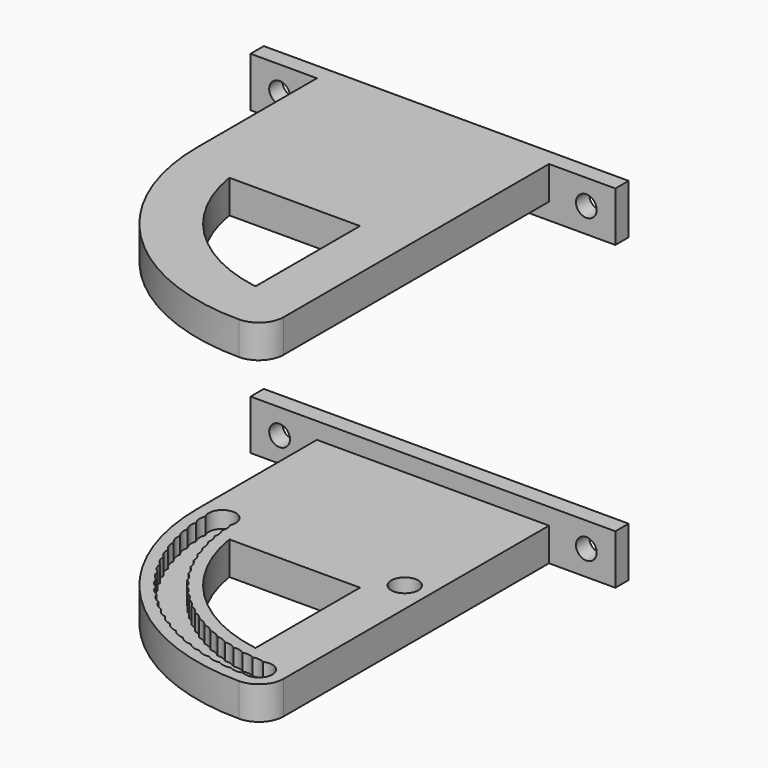
from build123d import *

# Parameters (mm, degrees)
F0_R          = 1.625
F1_DEPTH      = 2
F2_R          = 1.625
F3_DEPTH      = 2
F4_W          = 8
F4_H          = 2
F4_W_2        = 28
F5_DEPTH      = 2
F5_DEPTH_BACK = 4
F6_R          = 1.25
F7_DEPTH      = 25


with BuildPart() as f1:
    # F0 (on Top) → F1 (new body)
    with BuildSketch(Plane.XY):
        with BuildLine():
            Line((-25, 20), (-25, 0))
            ThreePointArc((-25, 0), (-17.6776695297, -17.6776695297), (0, -25))
            ThreePointArc((0, -25), (2.1213203436, -24.1213203436), (3, -22))
            Line((3, -22), (3, 20))
            Line((3, 20), (-25, 20))
        make_face()
        with BuildLine():
            ThreePointArc((-0.6717668116, -20.520353302), (1.6241299546, -22.0531685096), (-0.7671020315, -23.4325430092))
            ThreePointArc((-0.7671020315, -23.4325430092), (-1.5451489281, -23.5744170615), (-2.2980212458, -23.3322012626))
            ThreePointArc((-2.2980212458, -23.3322012626), (-3.0836812912, -23.42288485), (-3.8190999803, -23.1319474482))
            ThreePointArc((-3.8190999803, -23.1319474482), (-4.6090088576, -23.1710522495), (-5.3238247424, -22.8326390835))
            ThreePointArc((-5.3238247424, -22.8326390835), (-6.1145999405, -22.8199976461), (-6.8057520696, -22.435557853))
            ThreePointArc((-6.8057520696, -22.435557853), (-7.5940073678, -22.3712243093), (-8.2585361216, -21.9424041193))
            ThreePointArc((-8.2585361216, -21.9424041193), (-9.0408960896, -21.8266539556), (-9.675955854, -21.3552896425))
            ThreePointArc((-9.675955854, -21.3552896425), (-10.4490703064, -21.1886185187), (-11.0519416581, -20.676728537))
            ThreePointArc((-11.0519416581, -20.676728537), (-11.8125, -20.4598501644), (-12.3806013512, -19.9096265055))
            ThreePointArc((-12.3806013512, -19.9096265055), (-13.1253467551, -19.6434695906), (-13.6562454086, -19.0572683968))
            ThreePointArc((-13.6562454086, -19.0572683968), (-14.3819887603, -18.7429726644), (-14.8734113266, -18.123304139))
            ThreePointArc((-14.8734113266, -18.123304139), (-15.5770448817, -17.7622154517), (-16.026887014, -17.1117331106))
            ThreePointArc((-16.026887014, -17.1117331106), (-16.7053977055, -16.7053977055), (-17.1117331106, -16.026887014))
            ThreePointArc((-17.1117331106, -16.026887014), (-17.7622154517, -15.5770448817), (-18.123304139, -14.8734113266))
            ThreePointArc((-18.123304139, -14.8734113266), (-18.7429726644, -14.3819887603), (-19.0572683968, -13.6562454086))
            ThreePointArc((-19.0572683968, -13.6562454086), (-19.6434695906, -13.1253467551), (-19.9096265055, -12.3806013512))
            ThreePointArc((-19.9096265055, -12.3806013512), (-20.4598501644, -11.8125), (-20.676728537, -11.0519416581))
            ThreePointArc((-20.676728537, -11.0519416581), (-21.1886185187, -10.4490703064), (-21.3552896425, -9.675955854))
            ThreePointArc((-21.3552896425, -9.675955854), (-21.8266539556, -9.0408960896), (-21.9424041193, -8.2585361216))
            ThreePointArc((-21.9424041193, -8.2585361216), (-22.3712243093, -7.5940073678), (-22.435557853, -6.8057520696))
            ThreePointArc((-22.435557853, -6.8057520696), (-22.8199976461, -6.1145999405), (-22.8326390835, -5.3238247424))
            ThreePointArc((-22.8326390835, -5.3238247424), (-23.1710522495, -4.6090088576), (-23.1319474482, -3.8190999803))
            ThreePointArc((-23.1319474482, -3.8190999803), (-23.42288485, -3.0836812912), (-23.3322012626, -2.2980212458))
            ThreePointArc((-23.3322012626, -2.2980212458), (-23.5744170615, -1.5451489281), (-23.4325430092, -0.7671020315))
            ThreePointArc((-23.4325430092, -0.7671020315), (-22.0531685096, 1.6241299546), (-20.520353302, -0.6717668116))
            ThreePointArc((-20.520353302, -0.6717668116), (-20.331375561, -1.3325887581), (-20.4324819988, -2.0124238261))
            ThreePointArc((-20.4324819988, -2.0124238261), (-20.2006890505, -2.6594711665), (-20.2571156709, -3.3444633329))
            ThreePointArc((-20.2571156709, -3.3444633329), (-19.9835000882, -3.9749653111), (-19.9950052637, -4.6621813342))
            ThreePointArc((-19.9950052637, -4.6621813342), (-19.6807387106, -5.273438044), (-19.6472731743, -5.9599351593))
            ThreePointArc((-19.6472731743, -5.9599351593), (-19.2937013885, -6.5493291056), (-19.2154084448, -7.2321676271))
            ThreePointArc((-19.2154084448, -7.2321676271), (-18.8240454749, -7.7971749344), (-18.7012603864, -8.4734308428))
            ThreePointArc((-18.7012603864, -8.4734308428), (-18.2737821087, -9.0116320632), (-18.10703066, -9.6784095268))
            ThreePointArc((-18.10703066, -9.6784095268), (-17.6452676021, -10.1875), (-17.4352638484, -10.8419437753))
            ThreePointArc((-17.4352638484, -10.8419437753), (-16.9411933507, -11.3197434978), (-16.6888365603, -11.959051156))
            ThreePointArc((-16.6888365603, -11.959051156), (-16.1645743084, -12.4035141161), (-15.8709451119, -13.0249480438))
            ThreePointArc((-15.8709451119, -13.0249480438), (-15.3187360774, -13.4341709827), (-14.98509184, -14.0350701044))
            ThreePointArc((-14.98509184, -14.0350701044), (-14.4073006667, -14.4073006667), (-14.0350701044, -14.98509184))
            ThreePointArc((-14.0350701044, -14.98509184), (-13.4341709827, -15.3187360774), (-13.0249480438, -15.8709451119))
            ThreePointArc((-13.0249480438, -15.8709451119), (-12.4035141161, -16.1645743084), (-11.959051156, -16.6888365603))
            ThreePointArc((-11.959051156, -16.6888365603), (-11.3197434978, -16.9411933507), (-10.8419437753, -17.4352638484))
            ThreePointArc((-10.8419437753, -17.4352638484), (-10.1875, -17.6452676021), (-9.6784095268, -18.10703066))
            ThreePointArc((-9.6784095268, -18.10703066), (-9.0116320632, -18.2737821087), (-8.4734308428, -18.7012603864))
            ThreePointArc((-8.4734308428, -18.7012603864), (-7.7971749344, -18.8240454749), (-7.2321676271, -19.2154084448))
            ThreePointArc((-7.2321676271, -19.2154084448), (-6.5493291056, -19.2937013885), (-5.9599351593, -19.6472731743))
            ThreePointArc((-5.9599351593, -19.6472731743), (-5.273438044, -19.6807387106), (-4.6621813342, -19.9950052637))
            ThreePointArc((-4.6621813342, -19.9950052637), (-3.9749653111, -19.9835000882), (-3.3444633329, -20.2571156709))
            ThreePointArc((-3.3444633329, -20.2571156709), (-2.6594711665, -20.2006890505), (-2.0124238261, -20.4324819988))
            ThreePointArc((-2.0124238261, -20.4324819988), (-1.3325887581, -20.331375561), (-0.6717668116, -20.520353302))
        make_face(mode=Mode.SUBTRACT)
        with BuildLine():
            ThreePointArc((-3, -18.7616630393), (-13.4350288425, -13.4350288425), (-18.7616630393, -3))
            Line((-18.7616630393, -3), (-3, -3))
            Line((-3, -3), (-3, -18.7616630393))
        make_face(mode=Mode.SUBTRACT)
        Circle(F0_R, mode=Mode.SUBTRACT)
    extrude(amount=F1_DEPTH)

    # F2 (on face) → F3 (join)
    with BuildSketch(Plane(origin=(0, 0, 0), x_dir=(1, 0, 0), z_dir=(0, 0, -1))):
        with BuildLine():
            ThreePointArc((0, 25), (-17.6776695297, 17.6776695297), (-25, 0))
            Line((-25, 0), (-25, -20))
            Line((-25, -20), (3, -20))
            Line((3, -20), (3, 22))
            ThreePointArc((3, 22), (2.1213203436, 24.1213203436), (0, 25))
        make_face()
        Circle(F2_R, mode=Mode.SUBTRACT)
        with BuildLine():
            Line((-3, 18.7616630393), (-3, 3))
            Line((-3, 3), (-18.7616630393, 3))
            ThreePointArc((-18.7616630393, 3), (-13.4350288425, 13.4350288425), (-3, 18.7616630393))
        make_face(mode=Mode.SUBTRACT)
        with BuildLine():
            ThreePointArc((-2.2980212458, 23.3322012626), (-1.5451489281, 23.5744170615), (-0.7671020315, 23.4325430092))
            ThreePointArc((-0.7671020315, 23.4325430092), (1.6241299546, 22.0531685096), (-0.6717668116, 20.520353302))
            ThreePointArc((-0.6717668116, 20.520353302), (-1.3325887581, 20.331375561), (-2.0124238261, 20.4324819988))
            ThreePointArc((-2.0124238261, 20.4324819988), (-2.6594711665, 20.2006890505), (-3.3444633329, 20.2571156709))
            ThreePointArc((-3.3444633329, 20.2571156709), (-3.9749653111, 19.9835000882), (-4.6621813342, 19.9950052637))
            ThreePointArc((-4.6621813342, 19.9950052637), (-5.273438044, 19.6807387106), (-5.9599351593, 19.6472731743))
            ThreePointArc((-5.9599351593, 19.6472731743), (-6.5493291056, 19.2937013885), (-7.2321676271, 19.2154084448))
            ThreePointArc((-7.2321676271, 19.2154084448), (-7.7971749344, 18.8240454749), (-8.4734308428, 18.7012603864))
            ThreePointArc((-8.4734308428, 18.7012603864), (-9.0116320632, 18.2737821087), (-9.6784095268, 18.10703066))
            ThreePointArc((-9.6784095268, 18.10703066), (-10.1875, 17.6452676021), (-10.8419437753, 17.4352638484))
            ThreePointArc((-10.8419437753, 17.4352638484), (-11.3197434978, 16.9411933507), (-11.959051156, 16.6888365603))
            ThreePointArc((-11.959051156, 16.6888365603), (-12.4035141161, 16.1645743084), (-13.0249480438, 15.8709451119))
            ThreePointArc((-13.0249480438, 15.8709451119), (-13.4341709827, 15.3187360774), (-14.0350701044, 14.98509184))
            ThreePointArc((-14.0350701044, 14.98509184), (-14.4073006667, 14.4073006667), (-14.98509184, 14.0350701044))
            ThreePointArc((-14.98509184, 14.0350701044), (-15.3187360774, 13.4341709827), (-15.8709451119, 13.0249480438))
            ThreePointArc((-15.8709451119, 13.0249480438), (-16.1645743084, 12.4035141161), (-16.6888365603, 11.959051156))
            ThreePointArc((-16.6888365603, 11.959051156), (-16.9411933507, 11.3197434978), (-17.4352638484, 10.8419437753))
            ThreePointArc((-17.4352638484, 10.8419437753), (-17.6452676021, 10.1875), (-18.10703066, 9.6784095268))
            ThreePointArc((-18.10703066, 9.6784095268), (-18.2737821087, 9.0116320632), (-18.7012603864, 8.4734308428))
            ThreePointArc((-18.7012603864, 8.4734308428), (-18.8240454749, 7.7971749344), (-19.2154084448, 7.2321676271))
            ThreePointArc((-19.2154084448, 7.2321676271), (-19.2937013885, 6.5493291056), (-19.6472731743, 5.9599351593))
            ThreePointArc((-19.6472731743, 5.9599351593), (-19.6807387106, 5.273438044), (-19.9950052637, 4.6621813342))
            ThreePointArc((-19.9950052637, 4.6621813342), (-19.9835000882, 3.9749653111), (-20.2571156709, 3.3444633329))
            ThreePointArc((-20.2571156709, 3.3444633329), (-20.2006890505, 2.6594711665), (-20.4324819988, 2.0124238261))
            ThreePointArc((-20.4324819988, 2.0124238261), (-20.331375561, 1.3325887581), (-20.520353302, 0.6717668116))
            ThreePointArc((-20.520353302, 0.6717668116), (-22.0531685096, -1.6241299546), (-23.4325430092, 0.7671020315))
            ThreePointArc((-23.4325430092, 0.7671020315), (-23.5744170615, 1.5451489281), (-23.3322012626, 2.2980212458))
            ThreePointArc((-23.3322012626, 2.2980212458), (-23.42288485, 3.0836812912), (-23.1319474482, 3.8190999803))
            ThreePointArc((-23.1319474482, 3.8190999803), (-23.1710522495, 4.6090088576), (-22.8326390835, 5.3238247424))
            ThreePointArc((-22.8326390835, 5.3238247424), (-22.8199976461, 6.1145999405), (-22.435557853, 6.8057520696))
            ThreePointArc((-22.435557853, 6.8057520696), (-22.3712243093, 7.5940073678), (-21.9424041193, 8.2585361216))
            ThreePointArc((-21.9424041193, 8.2585361216), (-21.8266539556, 9.0408960896), (-21.3552896425, 9.675955854))
            ThreePointArc((-21.3552896425, 9.675955854), (-21.1886185187, 10.4490703064), (-20.676728537, 11.0519416581))
            ThreePointArc((-20.676728537, 11.0519416581), (-20.4598501644, 11.8125), (-19.9096265055, 12.3806013512))
            ThreePointArc((-19.9096265055, 12.3806013512), (-19.6434695906, 13.1253467551), (-19.0572683968, 13.6562454086))
            ThreePointArc((-19.0572683968, 13.6562454086), (-18.7429726644, 14.3819887603), (-18.123304139, 14.8734113266))
            ThreePointArc((-18.123304139, 14.8734113266), (-17.7622154517, 15.5770448817), (-17.1117331106, 16.026887014))
            ThreePointArc((-17.1117331106, 16.026887014), (-16.7053977055, 16.7053977055), (-16.026887014, 17.1117331106))
            ThreePointArc((-16.026887014, 17.1117331106), (-15.5770448817, 17.7622154517), (-14.8734113266, 18.123304139))
            ThreePointArc((-14.8734113266, 18.123304139), (-14.3819887603, 18.7429726644), (-13.6562454086, 19.0572683968))
            ThreePointArc((-13.6562454086, 19.0572683968), (-13.1253467551, 19.6434695906), (-12.3806013512, 19.9096265055))
            ThreePointArc((-12.3806013512, 19.9096265055), (-11.8125, 20.4598501644), (-11.0519416581, 20.676728537))
            ThreePointArc((-11.0519416581, 20.676728537), (-10.4490703064, 21.1886185187), (-9.675955854, 21.3552896425))
            ThreePointArc((-9.675955854, 21.3552896425), (-9.0408960896, 21.8266539556), (-8.2585361216, 21.9424041193))
            ThreePointArc((-8.2585361216, 21.9424041193), (-7.5940073678, 22.3712243093), (-6.8057520696, 22.435557853))
            ThreePointArc((-6.8057520696, 22.435557853), (-6.1145999405, 22.8199976461), (-5.3238247424, 22.8326390835))
            ThreePointArc((-5.3238247424, 22.8326390835), (-4.6090088576, 23.1710522495), (-3.8190999803, 23.1319474482))
            ThreePointArc((-3.8190999803, 23.1319474482), (-3.0836812912, 23.42288485), (-2.2980212458, 23.3322012626))
        make_face(mode=Mode.SUBTRACT)
        with BuildLine():
            ThreePointArc((-0.6717668116, 20.520353302), (1.6241299546, 22.0531685096), (-0.7671020315, 23.4325430092))
            ThreePointArc((-0.7671020315, 23.4325430092), (-1.5451489281, 23.5744170615), (-2.2980212458, 23.3322012626))
            ThreePointArc((-2.2980212458, 23.3322012626), (-3.0836812912, 23.42288485), (-3.8190999803, 23.1319474482))
            ThreePointArc((-3.8190999803, 23.1319474482), (-4.6090088576, 23.1710522495), (-5.3238247424, 22.8326390835))
            ThreePointArc((-5.3238247424, 22.8326390835), (-6.1145999405, 22.8199976461), (-6.8057520696, 22.435557853))
            ThreePointArc((-6.8057520696, 22.435557853), (-7.5940073678, 22.3712243093), (-8.2585361216, 21.9424041193))
            ThreePointArc((-8.2585361216, 21.9424041193), (-9.0408960896, 21.8266539556), (-9.675955854, 21.3552896425))
            ThreePointArc((-9.675955854, 21.3552896425), (-10.4490703064, 21.1886185187), (-11.0519416581, 20.676728537))
            ThreePointArc((-11.0519416581, 20.676728537), (-11.8125, 20.4598501644), (-12.3806013512, 19.9096265055))
            ThreePointArc((-12.3806013512, 19.9096265055), (-13.1253467551, 19.6434695906), (-13.6562454086, 19.0572683968))
            ThreePointArc((-13.6562454086, 19.0572683968), (-14.3819887603, 18.7429726644), (-14.8734113266, 18.123304139))
            ThreePointArc((-14.8734113266, 18.123304139), (-15.5770448817, 17.7622154517), (-16.026887014, 17.1117331106))
            ThreePointArc((-16.026887014, 17.1117331106), (-16.7053977055, 16.7053977055), (-17.1117331106, 16.026887014))
            ThreePointArc((-17.1117331106, 16.026887014), (-17.7622154517, 15.5770448817), (-18.123304139, 14.8734113266))
            ThreePointArc((-18.123304139, 14.8734113266), (-18.7429726644, 14.3819887603), (-19.0572683968, 13.6562454086))
            ThreePointArc((-19.0572683968, 13.6562454086), (-19.6434695906, 13.1253467551), (-19.9096265055, 12.3806013512))
            ThreePointArc((-19.9096265055, 12.3806013512), (-20.4598501644, 11.8125), (-20.676728537, 11.0519416581))
            ThreePointArc((-20.676728537, 11.0519416581), (-21.1886185187, 10.4490703064), (-21.3552896425, 9.675955854))
            ThreePointArc((-21.3552896425, 9.675955854), (-21.8266539556, 9.0408960896), (-21.9424041193, 8.2585361216))
            ThreePointArc((-21.9424041193, 8.2585361216), (-22.3712243093, 7.5940073678), (-22.435557853, 6.8057520696))
            ThreePointArc((-22.435557853, 6.8057520696), (-22.8199976461, 6.1145999405), (-22.8326390835, 5.3238247424))
            ThreePointArc((-22.8326390835, 5.3238247424), (-23.1710522495, 4.6090088576), (-23.1319474482, 3.8190999803))
            ThreePointArc((-23.1319474482, 3.8190999803), (-23.42288485, 3.0836812912), (-23.3322012626, 2.2980212458))
            ThreePointArc((-23.3322012626, 2.2980212458), (-23.5744170615, 1.5451489281), (-23.4325430092, 0.7671020315))
            ThreePointArc((-23.4325430092, 0.7671020315), (-22.0531685096, -1.6241299546), (-20.520353302, 0.6717668116))
            ThreePointArc((-20.520353302, 0.6717668116), (-20.331375561, 1.3325887581), (-20.4324819988, 2.0124238261))
            ThreePointArc((-20.4324819988, 2.0124238261), (-20.2006890505, 2.6594711665), (-20.2571156709, 3.3444633329))
            ThreePointArc((-20.2571156709, 3.3444633329), (-19.9835000882, 3.9749653111), (-19.9950052637, 4.6621813342))
            ThreePointArc((-19.9950052637, 4.6621813342), (-19.6807387106, 5.273438044), (-19.6472731743, 5.9599351593))
            ThreePointArc((-19.6472731743, 5.9599351593), (-19.2937013885, 6.5493291056), (-19.2154084448, 7.2321676271))
            ThreePointArc((-19.2154084448, 7.2321676271), (-18.8240454749, 7.7971749344), (-18.7012603864, 8.4734308428))
            ThreePointArc((-18.7012603864, 8.4734308428), (-18.2737821087, 9.0116320632), (-18.10703066, 9.6784095268))
            ThreePointArc((-18.10703066, 9.6784095268), (-17.6452676021, 10.1875), (-17.4352638484, 10.8419437753))
            ThreePointArc((-17.4352638484, 10.8419437753), (-16.9411933507, 11.3197434978), (-16.6888365603, 11.959051156))
            ThreePointArc((-16.6888365603, 11.959051156), (-16.1645743084, 12.4035141161), (-15.8709451119, 13.0249480438))
            ThreePointArc((-15.8709451119, 13.0249480438), (-15.3187360774, 13.4341709827), (-14.98509184, 14.0350701044))
            ThreePointArc((-14.98509184, 14.0350701044), (-14.4073006667, 14.4073006667), (-14.0350701044, 14.98509184))
            ThreePointArc((-14.0350701044, 14.98509184), (-13.4341709827, 15.3187360774), (-13.0249480438, 15.8709451119))
            ThreePointArc((-13.0249480438, 15.8709451119), (-12.4035141161, 16.1645743084), (-11.959051156, 16.6888365603))
            ThreePointArc((-11.959051156, 16.6888365603), (-11.3197434978, 16.9411933507), (-10.8419437753, 17.4352638484))
            ThreePointArc((-10.8419437753, 17.4352638484), (-10.1875, 17.6452676021), (-9.6784095268, 18.10703066))
            ThreePointArc((-9.6784095268, 18.10703066), (-9.0116320632, 18.2737821087), (-8.4734308428, 18.7012603864))
            ThreePointArc((-8.4734308428, 18.7012603864), (-7.7971749344, 18.8240454749), (-7.2321676271, 19.2154084448))
            ThreePointArc((-7.2321676271, 19.2154084448), (-6.5493291056, 19.2937013885), (-5.9599351593, 19.6472731743))
            ThreePointArc((-5.9599351593, 19.6472731743), (-5.273438044, 19.6807387106), (-4.6621813342, 19.9950052637))
            ThreePointArc((-4.6621813342, 19.9950052637), (-3.9749653111, 19.9835000882), (-3.3444633329, 20.2571156709))
            ThreePointArc((-3.3444633329, 20.2571156709), (-2.6594711665, 20.2006890505), (-2.0124238261, 20.4324819988))
            ThreePointArc((-2.0124238261, 20.4324819988), (-1.3325887581, 20.331375561), (-0.6717668116, 20.520353302))
        make_face()
        Circle(F2_R)
    extrude(amount=F3_DEPTH)

    # F4 (on face) → F5 (join, two sides)
    with BuildSketch(Plane.XY.offset(2)) as f5_sk:
        with Locations((-29, 19)):
            Rectangle(F4_W, F4_H)
        with Locations((-11, 19)):
            Rectangle(F4_W_2, F4_H)
        with Locations((7, 19)):
            Rectangle(F4_W, F4_H)
    extrude(amount=F5_DEPTH)
    extrude(f5_sk.sketch, amount=-F5_DEPTH_BACK)

    # F6 (on face) → F7 (cut)
    with BuildSketch(Plane.XZ.offset(-18)):
        with Locations((7.5, 1)):
            Circle(F6_R)
        with Locations((-29.5, 1)):
            Circle(F6_R)
    extrude(amount=-F7_DEPTH, mode=Mode.SUBTRACT)


with BuildPart() as f9_1:
    # F9: instance of F1
    add(f1.part.mirror(Plane.XY.offset(19.2)))


solid = Compound([f1.part, f9_1.part])
